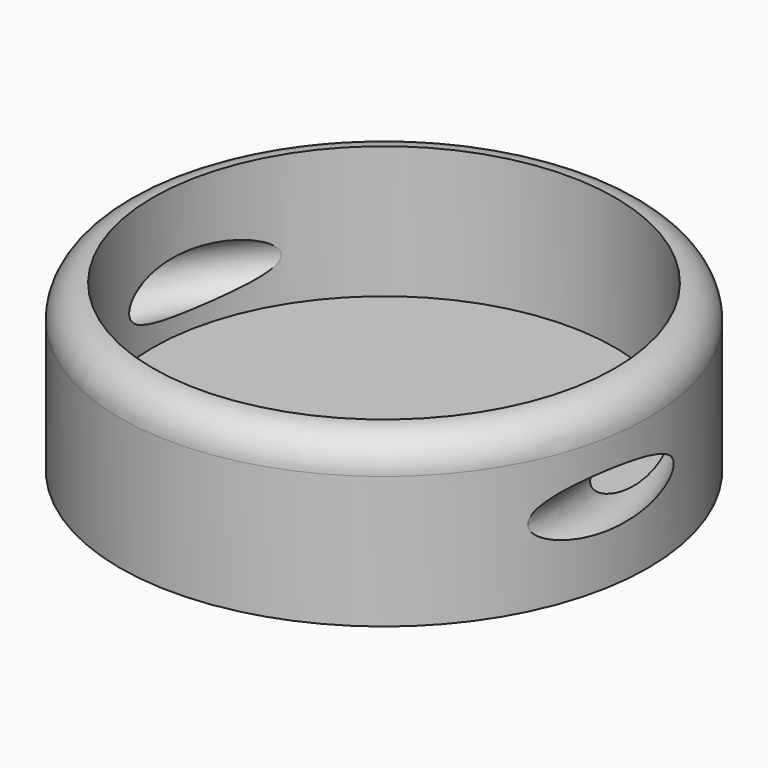
from build123d import *

# Parameters (mm, degrees)
F0_R         = 40
F1_DEPTH     = 25
F2_R         = 35
F3_DEPTH     = 20
F4_R         = 4.99999
F5_R         = 4.0430384516
F7_TEXT_SIZE = 20.366265542
F8_DEPTH     = 1


# Not quite as in the source:
# - a fillet or chamfer is up to 0.001 mm smaller than in the source, because OpenCascade refuses the exact size
# - Text() gives the source's letters only with a copy of the font that has no kerning and outlines rounded to 1/6400 em; it was checked with that copy


with BuildPart() as f1:
    # F0 (on Top) → F1 (new body)
    with BuildSketch(Plane.XY):
        with Locations((-1.2652061832, 14.1146601946)):
            Circle(F0_R)
    extrude(amount=F1_DEPTH)

    # F2 (on face) → F3 (cut)
    with BuildSketch(Plane.XY.offset(25)):
        with Locations((-1.2652061832, 14.1146601946)):
            Circle(F2_R)
    extrude(amount=-F3_DEPTH, mode=Mode.SUBTRACT)

    # F4 (radius 5 in the source; OpenCascade refuses exactly that, so slightly less here)
    f4_edges = [f1.edges().sort_by_distance(p)[0] for p in [
        (-41.265206, 14.11466, 25),
    ]]
    fillet(f4_edges, radius=F4_R)

    # F5 (on Front) → F6 (revolve, cut)
    with BuildSketch(Plane.XZ):
        with Locations((-41.1538481712, 11.6346161813)):
            Circle(F5_R)
    revolve(axis=Axis((-1.1538460385, 0, 14.903847321), (0, 0, -1)), mode=Mode.SUBTRACT)

    # F7 (on face) → F8 (cut)
    with BuildSketch(Plane(origin=(0, 0, 0), x_dir=(1, 0, 0), z_dir=(0, 0, -1))):
        with Locations((-30.3559303284, -21.9260295853)):
            Text('BORIS', F7_TEXT_SIZE, font='Open Sans', text_align=(TextAlign.LEFT, TextAlign.BOTTOM))
    extrude(amount=-F8_DEPTH, mode=Mode.SUBTRACT)


solid = f1.part
